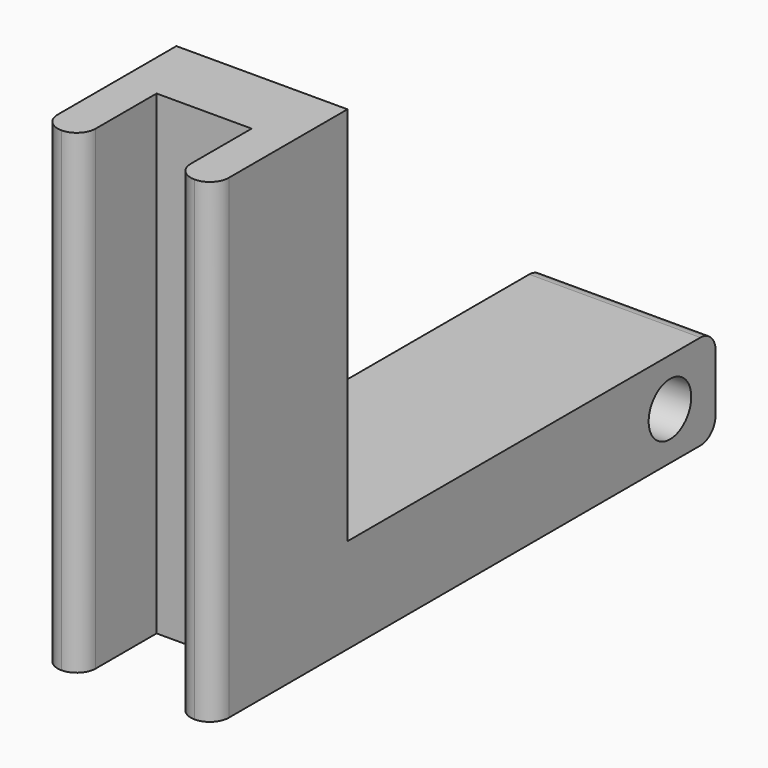
from build123d import *

# Parameters (mm, degrees)
F1_DEPTH = 25
F0_W     = 9
F0_H     = 24.2
F2_DEPTH = 5
F3_R     = 1.4
F4_DEPTH = 12.5
F5_R     = 0.99999


# Not quite as in the source:
# - a fillet or chamfer is up to 0.001 mm smaller than in the source, because OpenCascade refuses the exact size


with BuildPart() as f1:
    # F0 (on Top) → F1 (new body)
    with BuildSketch(Plane.XY):
        Polygon((-4.5, 8.8), (-4.5, 0), (-2.5, 0), (-2.5, 5), (2.5, 5), (2.5, 0), (4.5, 0), (4.5, 8.8), align=None)
    extrude(amount=F1_DEPTH)

    # F0 (on Top) → F2 (join)
    with BuildSketch(Plane.XY):
        with Locations((0, 20.9)):
            Rectangle(F0_W, F0_H)
    extrude(amount=F2_DEPTH)

    # F3 (on Right) → F4 (cut, symmetric)
    with BuildSketch(Plane.YZ):
        with Locations((30, 2.5)):
            Circle(F3_R)
    extrude(amount=F4_DEPTH, both=True, mode=Mode.SUBTRACT)

    # F5 (radius 1 in the source; OpenCascade refuses exactly that, so slightly less here)
    f5_edges = [f1.edges().sort_by_distance(p)[0] for p in [
        (0, 33, 5),
        (0, 33, 0),
        (-2.5, 0, 12.5),
        (2.5, 0, 12.5),
        (-4.5, 0, 12.5),
        (4.5, 0, 12.5),
    ]]
    fillet(f5_edges, radius=F5_R)


solid = f1.part
